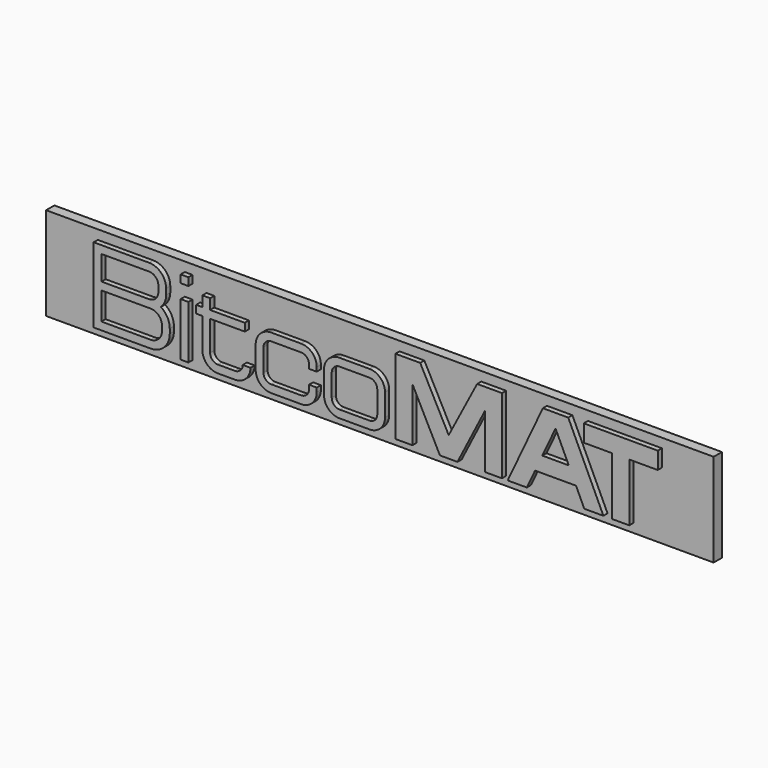
from build123d import *

# Parameters (mm, degrees)
F0_W     = 129
F0_H     = 18
F0_W_2   = 1.5
F0_H_2   = 10.3
F0_R     = 2.1
F0_H_3   = 1.5
F1_DEPTH = 2
F2_DEPTH = 1
F3_R     = 2.1
F4_DEPTH = 2


with BuildPart() as f1:
    # F0 (on Front) → F1 (new body)
    with BuildSketch(Plane.XZ):
        with Locations((64.5, 9)):
            Rectangle(F0_W, F0_H)
        with Locations((27.55, 6.85)):
            Rectangle(F0_W_2, F0_H_2, mode=Mode.SUBTRACT)
        with BuildLine():
            Line((10, 1.7), (10, 16.2))
            Line((10, 16.2), (20.7, 16.2))
            ThreePointArc((20.7, 16.2), (23.0334523779, 15.2334523779), (24, 12.9))
            Line((24, 12.9), (24, 11.8))
            ThreePointArc((24, 11.8), (23.7362385725, 10.5072295908), (22.9871179813, 9.4211155263))
            ThreePointArc((22.9871179813, 9.4211155263), (24.2436350389, 8.0801212696), (24.7, 6.3))
            Line((24.7, 6.3), (24.7, 5.4))
            ThreePointArc((24.7, 5.4), (23.6162950904, 2.7837049096), (21, 1.7))
            Line((21, 1.7), (10, 1.7))
        make_face(mode=Mode.SUBTRACT)
        with BuildLine():
            Line((32.5, 10.5), (32.5, 4.7))
            ThreePointArc((32.5, 4.7), (32.9393398282, 3.6393398282), (34, 3.2))
            Line((34, 3.2), (37.3, 3.2))
            ThreePointArc((37.3, 3.2), (38.3606601718, 3.6393398282), (38.8, 4.7))
            Line((38.8, 4.7), (40.3, 4.7))
            ThreePointArc((40.3, 4.7), (39.4213203436, 2.5786796564), (37.3, 1.7))
            Line((37.3, 1.7), (34, 1.7))
            ThreePointArc((34, 1.7), (31.8786796564, 2.5786796564), (31, 4.7))
            Line((31, 4.7), (31, 10.5))
            Line((31, 10.5), (29.8, 10.5))
            Line((29.8, 10.5), (29.8, 12))
            Line((29.8, 12), (31, 12))
            Line((31, 12), (31, 14))
            Line((31, 14), (32.5, 14))
            Line((32.5, 14), (32.5, 12))
            Line((32.5, 12), (39.2, 12))
            Line((39.2, 12), (39.2, 10.5))
            Line((39.2, 10.5), (32.5, 10.5))
        make_face(mode=Mode.SUBTRACT)
        with BuildLine():
            Line((50.1, 10.5), (44.3, 10.5))
            ThreePointArc((44.3, 10.5), (43.2393398282, 10.0606601718), (42.8, 9))
            Line((42.8, 9), (42.8, 4.7))
            ThreePointArc((42.8, 4.7), (43.2393398282, 3.6393398282), (44.3, 3.2))
            Line((44.3, 3.2), (50.1, 3.2))
            ThreePointArc((50.1, 3.2), (51.1606601718, 3.6393398282), (51.6, 4.7))
            Line((51.6, 4.7), (51.6, 5.5))
            Line((51.6, 5.5), (53.1, 5.5))
            Line((53.1, 5.5), (53.1, 4.7))
            ThreePointArc((53.1, 4.7), (52.2213203436, 2.5786796564), (50.1, 1.7))
            Line((50.1, 1.7), (44.3, 1.7))
            ThreePointArc((44.3, 1.7), (42.1786796564, 2.5786796564), (41.3, 4.7))
            Line((41.3, 4.7), (41.3, 9))
            ThreePointArc((41.3, 9), (42.1786796564, 11.1213203436), (44.3, 12))
            Line((44.3, 12), (50.1, 12))
            ThreePointArc((50.1, 12), (52.2213203436, 11.1213203436), (53.1, 9))
            Line((53.1, 9), (53.1, 8.2))
            Line((53.1, 8.2), (51.6, 8.2))
            Line((51.6, 8.2), (51.6, 9))
            ThreePointArc((51.6, 9), (51.1606601718, 10.0606601718), (50.1, 10.5))
        make_face(mode=Mode.SUBTRACT)
        with BuildLine():
            ThreePointArc((54.5, 9), (55.3786796564, 11.1213203436), (57.5, 12))
            Line((57.5, 12), (63.3, 12))
            ThreePointArc((63.3, 12), (65.4213203436, 11.1213203436), (66.3, 9))
            Line((66.3, 9), (66.3, 4.7))
            ThreePointArc((66.3, 4.7), (65.4213203436, 2.5786796564), (63.3, 1.7))
            Line((63.3, 1.7), (57.5, 1.7))
            ThreePointArc((57.5, 1.7), (55.3786796564, 2.5786796564), (54.5, 4.7))
            Line((54.5, 4.7), (54.5, 9))
        make_face(mode=Mode.SUBTRACT)
        Polygon((71.6, 12.1), (71.6, 1.7), (68.3, 1.7), (68.3, 16.2), (73.1, 16.2), (78.6, 5.7), (84.1, 16.2), (88.9, 16.2), (88.9, 1.7), (85.6, 1.7), (85.6, 12.1), (80.3, 1.7), (76.9, 1.7), align=None, mode=Mode.SUBTRACT)
        Polygon((93.7, 1.7), (90, 1.7), (96.8, 16.2), (101.7, 16.2), (108.5, 1.7), (104.8, 1.7), (103.2055172414, 5.1), (95.2944827586, 5.1), align=None, mode=Mode.SUBTRACT)
        Polygon((104.7, 12.9), (104.7, 16.2), (119, 16.2), (119, 12.9), (113.5, 12.9), (113.5, 1.7), (110.2, 1.7), (110.2, 12.9), align=None, mode=Mode.SUBTRACT)
        with Locations((5, 9)):
            Circle(F0_R, mode=Mode.SUBTRACT)
        with Locations((27.55, 15.45)):
            Rectangle(F0_W_2, F0_H_3, mode=Mode.SUBTRACT)
        with Locations((124, 9)):
            Circle(F0_R, mode=Mode.SUBTRACT)
        with BuildLine():
            Line((20.7, 16.2), (10, 16.2))
            Line((10, 16.2), (10, 1.7))
            Line((10, 1.7), (21, 1.7))
            ThreePointArc((21, 1.7), (23.6162950904, 2.7837049096), (24.7, 5.4))
            Line((24.7, 5.4), (24.7, 6.3))
            ThreePointArc((24.7, 6.3), (24.2436350389, 8.0801212696), (22.9871179813, 9.4211155263))
            ThreePointArc((22.9871179813, 9.4211155263), (23.7362385725, 10.5072295908), (24, 11.8))
            Line((24, 11.8), (24, 12.9))
            ThreePointArc((24, 12.9), (23.0334523779, 15.2334523779), (20.7, 16.2))
        make_face()
        with BuildLine():
            Line((11.5, 8.5), (21, 8.5))
            ThreePointArc((21, 8.5), (22.5556349186, 7.8556349186), (23.2, 6.3))
            Line((23.2, 6.3), (23.2, 5.4))
            ThreePointArc((23.2, 5.4), (22.5556349186, 3.8443650814), (21, 3.2))
            Line((21, 3.2), (11.5, 3.2))
            Line((11.5, 3.2), (11.5, 8.5))
        make_face(mode=Mode.SUBTRACT)
        with BuildLine():
            Line((11.5, 14.7), (20.7, 14.7))
            ThreePointArc((20.7, 14.7), (21.9727922061, 14.1727922061), (22.5, 12.9))
            Line((22.5, 12.9), (22.5, 11.8))
            ThreePointArc((22.5, 11.8), (21.9727922061, 10.5272077939), (20.7, 10))
            Line((20.7, 10), (11.5, 10))
            Line((11.5, 10), (11.5, 14.7))
        make_face(mode=Mode.SUBTRACT)
        Polygon((68.3, 1.7), (71.6, 1.7), (71.6, 12.1), (76.9, 1.7), (80.3, 1.7), (85.6, 12.1), (85.6, 1.7), (88.9, 1.7), (88.9, 16.2), (84.1, 16.2), (78.6, 5.7), (73.1, 16.2), (68.3, 16.2), align=None)
        Polygon((96.8, 16.2), (90, 1.7), (93.7, 1.7), (95.2944827586, 5.1), (103.2055172414, 5.1), (104.8, 1.7), (108.5, 1.7), (101.7, 16.2), align=None)
        Polygon((99.25, 13.5492647059), (101.8055172414, 8.1), (96.6944827586, 8.1), align=None, mode=Mode.SUBTRACT)
        with BuildLine():
            Line((63.3, 12), (57.5, 12))
            ThreePointArc((57.5, 12), (55.3786796564, 11.1213203436), (54.5, 9))
            Line((54.5, 9), (54.5, 4.7))
            ThreePointArc((54.5, 4.7), (55.3786796564, 2.5786796564), (57.5, 1.7))
            Line((57.5, 1.7), (63.3, 1.7))
            ThreePointArc((63.3, 1.7), (65.4213203436, 2.5786796564), (66.3, 4.7))
            Line((66.3, 4.7), (66.3, 9))
            ThreePointArc((66.3, 9), (65.4213203436, 11.1213203436), (63.3, 12))
        make_face()
        with BuildLine():
            ThreePointArc((56, 9), (56.4393398282, 10.0606601718), (57.5, 10.5))
            Line((57.5, 10.5), (63.3, 10.5))
            ThreePointArc((63.3, 10.5), (64.3606601718, 10.0606601718), (64.8, 9))
            Line((64.8, 9), (64.8, 4.7))
            ThreePointArc((64.8, 4.7), (64.3606601718, 3.6393398282), (63.3, 3.2))
            Line((63.3, 3.2), (57.5, 3.2))
            ThreePointArc((57.5, 3.2), (56.4393398282, 3.6393398282), (56, 4.7))
            Line((56, 4.7), (56, 9))
        make_face(mode=Mode.SUBTRACT)
        Polygon((119, 16.2), (104.7, 16.2), (104.7, 12.9), (110.2, 12.9), (110.2, 1.7), (113.5, 1.7), (113.5, 12.9), (119, 12.9), align=None)
        with BuildLine():
            Line((63.3, 10.5), (57.5, 10.5))
            ThreePointArc((57.5, 10.5), (56.4393398282, 10.0606601718), (56, 9))
            Line((56, 9), (56, 4.7))
            ThreePointArc((56, 4.7), (56.4393398282, 3.6393398282), (57.5, 3.2))
            Line((57.5, 3.2), (63.3, 3.2))
            ThreePointArc((63.3, 3.2), (64.3606601718, 3.6393398282), (64.8, 4.7))
            Line((64.8, 4.7), (64.8, 9))
            ThreePointArc((64.8, 9), (64.3606601718, 10.0606601718), (63.3, 10.5))
        make_face()
        with BuildLine():
            ThreePointArc((23.2, 6.3), (22.5556349186, 7.8556349186), (21, 8.5))
            Line((21, 8.5), (11.5, 8.5))
            Line((11.5, 8.5), (11.5, 3.2))
            Line((11.5, 3.2), (21, 3.2))
            ThreePointArc((21, 3.2), (22.5556349186, 3.8443650814), (23.2, 5.4))
            Line((23.2, 5.4), (23.2, 6.3))
        make_face()
        with BuildLine():
            ThreePointArc((22.5, 12.9), (21.9727922061, 14.1727922061), (20.7, 14.7))
            Line((20.7, 14.7), (11.5, 14.7))
            Line((11.5, 14.7), (11.5, 10))
            Line((11.5, 10), (20.7, 10))
            ThreePointArc((20.7, 10), (21.9727922061, 10.5272077939), (22.5, 11.8))
            Line((22.5, 11.8), (22.5, 12.9))
        make_face()
        with BuildLine():
            ThreePointArc((42.8, 9), (43.2393398282, 10.0606601718), (44.3, 10.5))
            Line((44.3, 10.5), (50.1, 10.5))
            ThreePointArc((50.1, 10.5), (51.1606601718, 10.0606601718), (51.6, 9))
            Line((51.6, 9), (51.6, 8.2))
            Line((51.6, 8.2), (53.1, 8.2))
            Line((53.1, 8.2), (53.1, 9))
            ThreePointArc((53.1, 9), (52.2213203436, 11.1213203436), (50.1, 12))
            Line((50.1, 12), (44.3, 12))
            ThreePointArc((44.3, 12), (42.1786796564, 11.1213203436), (41.3, 9))
            Line((41.3, 9), (41.3, 4.7))
            ThreePointArc((41.3, 4.7), (42.1786796564, 2.5786796564), (44.3, 1.7))
            Line((44.3, 1.7), (50.1, 1.7))
            ThreePointArc((50.1, 1.7), (52.2213203436, 2.5786796564), (53.1, 4.7))
            Line((53.1, 4.7), (53.1, 5.5))
            Line((53.1, 5.5), (51.6, 5.5))
            Line((51.6, 5.5), (51.6, 4.7))
            ThreePointArc((51.6, 4.7), (51.1606601718, 3.6393398282), (50.1, 3.2))
            Line((50.1, 3.2), (44.3, 3.2))
            ThreePointArc((44.3, 3.2), (43.2393398282, 3.6393398282), (42.8, 4.7))
            Line((42.8, 4.7), (42.8, 9))
        make_face()
        with BuildLine():
            ThreePointArc((34, 3.2), (32.9393398282, 3.6393398282), (32.5, 4.7))
            Line((32.5, 4.7), (32.5, 10.5))
            Line((32.5, 10.5), (39.2, 10.5))
            Line((39.2, 10.5), (39.2, 12))
            Line((39.2, 12), (32.5, 12))
            Line((32.5, 12), (32.5, 14))
            Line((32.5, 14), (31, 14))
            Line((31, 14), (31, 12))
            Line((31, 12), (29.8, 12))
            Line((29.8, 12), (29.8, 10.5))
            Line((29.8, 10.5), (31, 10.5))
            Line((31, 10.5), (31, 4.7))
            ThreePointArc((31, 4.7), (31.8786796564, 2.5786796564), (34, 1.7))
            Line((34, 1.7), (37.3, 1.7))
            ThreePointArc((37.3, 1.7), (39.4213203436, 2.5786796564), (40.3, 4.7))
            Line((40.3, 4.7), (38.8, 4.7))
            ThreePointArc((38.8, 4.7), (38.3606601718, 3.6393398282), (37.3, 3.2))
            Line((37.3, 3.2), (34, 3.2))
        make_face()
        with Locations((27.55, 6.85)):
            Rectangle(F0_W_2, F0_H_2)
        Polygon((96.6944827586, 8.1), (101.8055172414, 8.1), (99.25, 13.5492647059), align=None)
        with Locations((27.55, 15.45)):
            Rectangle(F0_W_2, F0_H_3)
    extrude(amount=-F1_DEPTH)

    # F0 (on Front) → F2 (join)
    with BuildSketch(Plane.XZ):
        with BuildLine():
            Line((20.7, 16.2), (10, 16.2))
            Line((10, 16.2), (10, 1.7))
            Line((10, 1.7), (21, 1.7))
            ThreePointArc((21, 1.7), (23.6162950904, 2.7837049096), (24.7, 5.4))
            Line((24.7, 5.4), (24.7, 6.3))
            ThreePointArc((24.7, 6.3), (24.2436350389, 8.0801212696), (22.9871179813, 9.4211155263))
            ThreePointArc((22.9871179813, 9.4211155263), (23.7362385725, 10.5072295908), (24, 11.8))
            Line((24, 11.8), (24, 12.9))
            ThreePointArc((24, 12.9), (23.0334523779, 15.2334523779), (20.7, 16.2))
        make_face()
        with BuildLine():
            Line((11.5, 8.5), (21, 8.5))
            ThreePointArc((21, 8.5), (22.5556349186, 7.8556349186), (23.2, 6.3))
            Line((23.2, 6.3), (23.2, 5.4))
            ThreePointArc((23.2, 5.4), (22.5556349186, 3.8443650814), (21, 3.2))
            Line((21, 3.2), (11.5, 3.2))
            Line((11.5, 3.2), (11.5, 8.5))
        make_face(mode=Mode.SUBTRACT)
        with BuildLine():
            Line((11.5, 14.7), (20.7, 14.7))
            ThreePointArc((20.7, 14.7), (21.9727922061, 14.1727922061), (22.5, 12.9))
            Line((22.5, 12.9), (22.5, 11.8))
            ThreePointArc((22.5, 11.8), (21.9727922061, 10.5272077939), (20.7, 10))
            Line((20.7, 10), (11.5, 10))
            Line((11.5, 10), (11.5, 14.7))
        make_face(mode=Mode.SUBTRACT)
        with Locations((27.55, 6.85)):
            Rectangle(F0_W_2, F0_H_2)
        with Locations((27.55, 15.45)):
            Rectangle(F0_W_2, F0_H_3)
        with BuildLine():
            ThreePointArc((34, 3.2), (32.9393398282, 3.6393398282), (32.5, 4.7))
            Line((32.5, 4.7), (32.5, 10.5))
            Line((32.5, 10.5), (39.2, 10.5))
            Line((39.2, 10.5), (39.2, 12))
            Line((39.2, 12), (32.5, 12))
            Line((32.5, 12), (32.5, 14))
            Line((32.5, 14), (31, 14))
            Line((31, 14), (31, 12))
            Line((31, 12), (29.8, 12))
            Line((29.8, 12), (29.8, 10.5))
            Line((29.8, 10.5), (31, 10.5))
            Line((31, 10.5), (31, 4.7))
            ThreePointArc((31, 4.7), (31.8786796564, 2.5786796564), (34, 1.7))
            Line((34, 1.7), (37.3, 1.7))
            ThreePointArc((37.3, 1.7), (39.4213203436, 2.5786796564), (40.3, 4.7))
            Line((40.3, 4.7), (38.8, 4.7))
            ThreePointArc((38.8, 4.7), (38.3606601718, 3.6393398282), (37.3, 3.2))
            Line((37.3, 3.2), (34, 3.2))
        make_face()
        with BuildLine():
            ThreePointArc((42.8, 9), (43.2393398282, 10.0606601718), (44.3, 10.5))
            Line((44.3, 10.5), (50.1, 10.5))
            ThreePointArc((50.1, 10.5), (51.1606601718, 10.0606601718), (51.6, 9))
            Line((51.6, 9), (51.6, 8.2))
            Line((51.6, 8.2), (53.1, 8.2))
            Line((53.1, 8.2), (53.1, 9))
            ThreePointArc((53.1, 9), (52.2213203436, 11.1213203436), (50.1, 12))
            Line((50.1, 12), (44.3, 12))
            ThreePointArc((44.3, 12), (42.1786796564, 11.1213203436), (41.3, 9))
            Line((41.3, 9), (41.3, 4.7))
            ThreePointArc((41.3, 4.7), (42.1786796564, 2.5786796564), (44.3, 1.7))
            Line((44.3, 1.7), (50.1, 1.7))
            ThreePointArc((50.1, 1.7), (52.2213203436, 2.5786796564), (53.1, 4.7))
            Line((53.1, 4.7), (53.1, 5.5))
            Line((53.1, 5.5), (51.6, 5.5))
            Line((51.6, 5.5), (51.6, 4.7))
            ThreePointArc((51.6, 4.7), (51.1606601718, 3.6393398282), (50.1, 3.2))
            Line((50.1, 3.2), (44.3, 3.2))
            ThreePointArc((44.3, 3.2), (43.2393398282, 3.6393398282), (42.8, 4.7))
            Line((42.8, 4.7), (42.8, 9))
        make_face()
        with BuildLine():
            Line((63.3, 12), (57.5, 12))
            ThreePointArc((57.5, 12), (55.3786796564, 11.1213203436), (54.5, 9))
            Line((54.5, 9), (54.5, 4.7))
            ThreePointArc((54.5, 4.7), (55.3786796564, 2.5786796564), (57.5, 1.7))
            Line((57.5, 1.7), (63.3, 1.7))
            ThreePointArc((63.3, 1.7), (65.4213203436, 2.5786796564), (66.3, 4.7))
            Line((66.3, 4.7), (66.3, 9))
            ThreePointArc((66.3, 9), (65.4213203436, 11.1213203436), (63.3, 12))
        make_face()
        with BuildLine():
            ThreePointArc((56, 9), (56.4393398282, 10.0606601718), (57.5, 10.5))
            Line((57.5, 10.5), (63.3, 10.5))
            ThreePointArc((63.3, 10.5), (64.3606601718, 10.0606601718), (64.8, 9))
            Line((64.8, 9), (64.8, 4.7))
            ThreePointArc((64.8, 4.7), (64.3606601718, 3.6393398282), (63.3, 3.2))
            Line((63.3, 3.2), (57.5, 3.2))
            ThreePointArc((57.5, 3.2), (56.4393398282, 3.6393398282), (56, 4.7))
            Line((56, 4.7), (56, 9))
        make_face(mode=Mode.SUBTRACT)
        Polygon((68.3, 1.7), (71.6, 1.7), (71.6, 12.1), (76.9, 1.7), (80.3, 1.7), (85.6, 12.1), (85.6, 1.7), (88.9, 1.7), (88.9, 16.2), (84.1, 16.2), (78.6, 5.7), (73.1, 16.2), (68.3, 16.2), align=None)
        Polygon((96.8, 16.2), (90, 1.7), (93.7, 1.7), (95.2944827586, 5.1), (103.2055172414, 5.1), (104.8, 1.7), (108.5, 1.7), (101.7, 16.2), align=None)
        Polygon((99.25, 13.5492647059), (101.8055172414, 8.1), (96.6944827586, 8.1), align=None, mode=Mode.SUBTRACT)
        Polygon((119, 16.2), (104.7, 16.2), (104.7, 12.9), (110.2, 12.9), (110.2, 1.7), (113.5, 1.7), (113.5, 12.9), (119, 12.9), align=None)
    extrude(amount=F2_DEPTH)

    # F3 (on face) → F4 (join, through all)
    with BuildSketch(Plane.XZ):
        with Locations((5, 9)):
            Circle(F3_R)
        with Locations((124, 9)):
            Circle(F3_R)
    extrude(amount=-F4_DEPTH)


solid = f1.part
